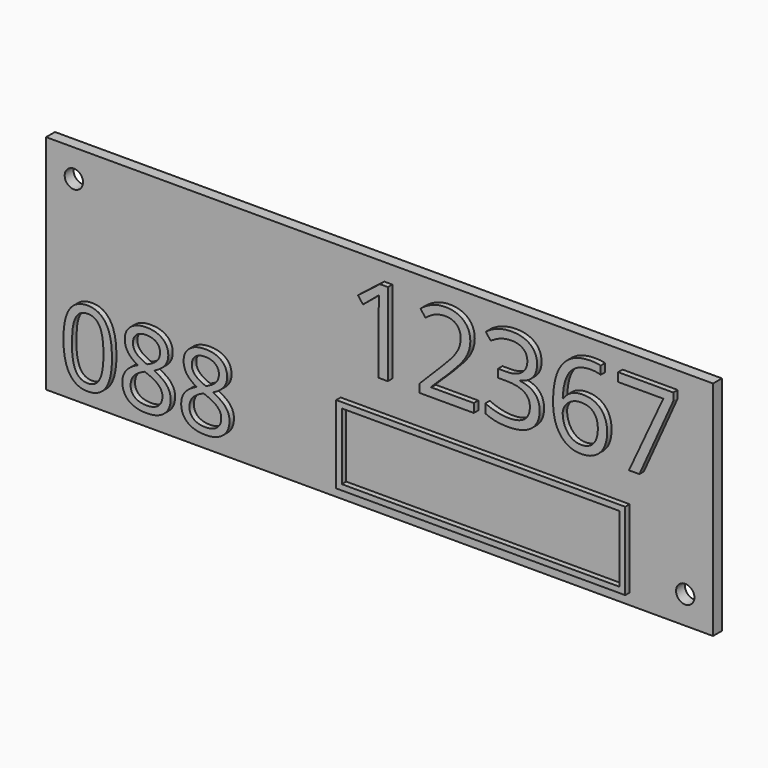
from build123d import *

# Parameters (mm, degrees)
F0_W         = 120
F0_H         = 40
F1_DEPTH     = 2
F3_D         = 3.3
F4_TEXT_SIZE = 20.8865923307
F5_DEPTH     = 1
F6_TEXT_SIZE = 18.5155049272
F7_DEPTH     = 1
F8_W         = 52
F8_H         = 14
F8_W_2       = 49.99999962
F8_H_2       = 11.99999962
F9_DEPTH     = 1


# Not quite as in the source:
# - Text() gives the source's letters only with a copy of the font that has no kerning and outlines rounded to 1/6400 em; it was checked with that copy


with BuildPart() as f1:
    # F0 (on Front) → F1 (new body)
    with BuildSketch(Plane.XZ):
        Rectangle(F0_W, F0_H)
    extrude(amount=F1_DEPTH)

    # F3 (through all)
    with Locations(Plane.XZ.offset(2)):
        with Locations((-55, 15), (55, -15)):
            Hole(F3_D / 2)

    # F4 (on face) → F5 (join)
    with BuildSketch(Plane.XZ.offset(2)):
        with Locations((-5, 2)):
            Text('12367', F4_TEXT_SIZE, font='Open Sans', text_align=(TextAlign.LEFT, TextAlign.BOTTOM))
    extrude(amount=F5_DEPTH)

    # F6 (on face) → F7 (join)
    with BuildSketch(Plane.XZ.offset(2)):
        with Locations((-57, -17)):
            Text('088', F6_TEXT_SIZE, font='Open Sans', text_align=(TextAlign.LEFT, TextAlign.BOTTOM))
    extrude(amount=F7_DEPTH)

    # F8 (on face) → F9 (join)
    with BuildSketch(Plane.XZ.offset(2)):
        with Locations((19, -11)):
            Rectangle(F8_W, F8_H)
        with Locations((19, -11)):
            Rectangle(F8_W_2, F8_H_2, mode=Mode.SUBTRACT)
    extrude(amount=F9_DEPTH)


solid = f1.part
